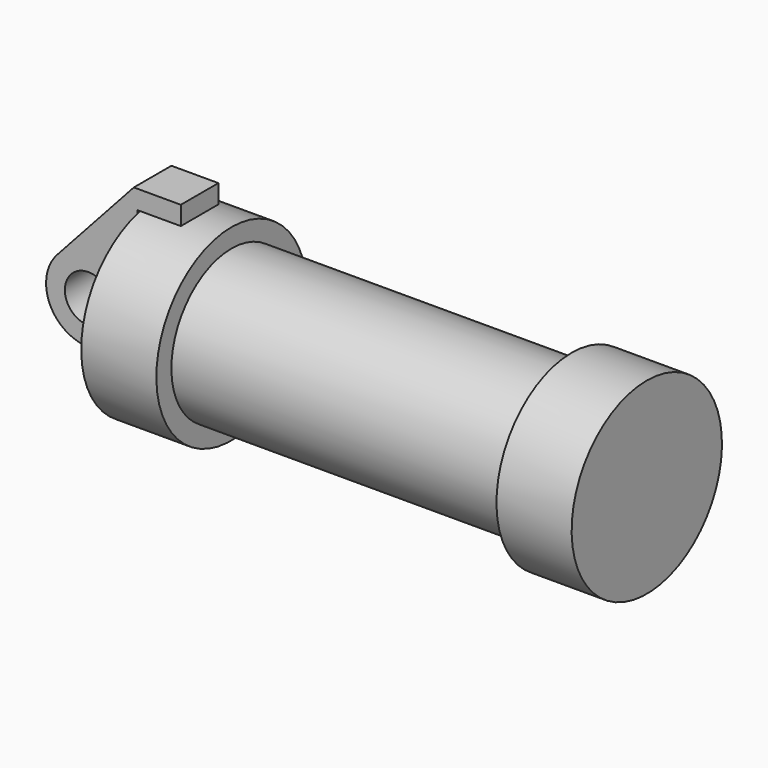
from build123d import *

# Parameters (mm, degrees)
F0_W     = 5.842
F0_H     = 12.7
F0_R     = 3.175
F2_DEPTH = 6.35
F4_DEPTH = 3.175


# Not quite as in the source:
# - a feature of the source that left no trace in its solid (it failed there, or was rolled back) is left out


with BuildPart() as f1:
    # F0 (on Front) → F1 (revolve)
    with BuildSketch(Plane.XZ):
        with Locations((2.921, 6.35)):
            Rectangle(F0_W, F0_H)
        Polygon((5.842, 12.7), (5.842, 0), (66.294, 0), (66.294, 12.7), (56.134, 12.7), (56.134, 10.16), (10.16, 10.16), (10.16, 12.7), align=None)
    revolve(axis=Axis((33.147, 0, 0), (-1, 0, 0)))


with BuildPart() as f2:
    # F0 (on Front) → F2 (new body)
    with BuildSketch(Plane.XZ):
        with BuildLine():
            Line((-0.9398, 0), (0, 0))
            Line((0, 0), (0, 12.7))
            Line((0, 12.7), (5.842, 12.7))
            Line((5.842, 12.7), (5.842, 15.24))
            Line((5.842, 15.24), (-0.508, 15.24))
            Line((-0.508, 15.24), (-10.8806298187, 3.8475430269))
            ThreePointArc((-10.8806298187, 3.8475430269), (-4.5919612295, 5.3297205562), (-0.9398, 0))
        make_face()
        with BuildLine():
            ThreePointArc((-8.1826630726, -5.5069827884), (-3.1957909266, -4.5493385486), (-0.9398, 0))
            ThreePointArc((-0.9398, 0), (-4.5919612295, 5.3297205562), (-10.8806298187, 3.8475430269))
            ThreePointArc((-10.8806298187, 3.8475430269), (-12.1459778134, -1.5837270034), (-8.1826630726, -5.5069827884))
        make_face()
        with Locations((-6.6548, 0)):
            Circle(F0_R, mode=Mode.SUBTRACT)
        with BuildLine():
            Line((5.842, 0), (0, 0))
            Line((0, 0), (-0.9398, 0))
            ThreePointArc((-0.9398, 0), (-3.1957909266, -4.5493385486), (-8.1826630726, -5.5069827884))
            Line((-8.1826630726, -5.5069827884), (5.842, -9.398))
            Line((5.842, -9.398), (5.842, 0))
        make_face()
    extrude(amount=F2_DEPTH)


with BuildPart() as f4:
    # F0 (on Front) → F4 (new body, symmetric)
    with BuildSketch(Plane.XZ):
        with BuildLine():
            ThreePointArc((-8.1826630726, -5.5069827884), (-3.1957909266, -4.5493385486), (-0.9398, 0))
            ThreePointArc((-0.9398, 0), (-4.5919612295, 5.3297205562), (-10.8806298187, 3.8475430269))
            ThreePointArc((-10.8806298187, 3.8475430269), (-12.1459778134, -1.5837270034), (-8.1826630726, -5.5069827884))
        make_face()
        with Locations((-6.6548, 0)):
            Circle(F0_R, mode=Mode.SUBTRACT)
        with BuildLine():
            Line((-0.9398, 0), (0, 0))
            Line((0, 0), (0, 12.7))
            Line((0, 12.7), (5.842, 12.7))
            Line((5.842, 12.7), (5.842, 15.24))
            Line((5.842, 15.24), (-0.508, 15.24))
            Line((-0.508, 15.24), (-10.8806298187, 3.8475430269))
            ThreePointArc((-10.8806298187, 3.8475430269), (-4.5919612295, 5.3297205562), (-0.9398, 0))
        make_face()
        with BuildLine():
            Line((5.842, 0), (0, 0))
            Line((0, 0), (-0.9398, 0))
            ThreePointArc((-0.9398, 0), (-3.1957909266, -4.5493385486), (-8.1826630726, -5.5069827884))
            Line((-8.1826630726, -5.5069827884), (5.842, -9.398))
            Line((5.842, -9.398), (5.842, 0))
        make_face()
    extrude(amount=F4_DEPTH, both=True)


solid = Compound([f1.part, f4.part])
